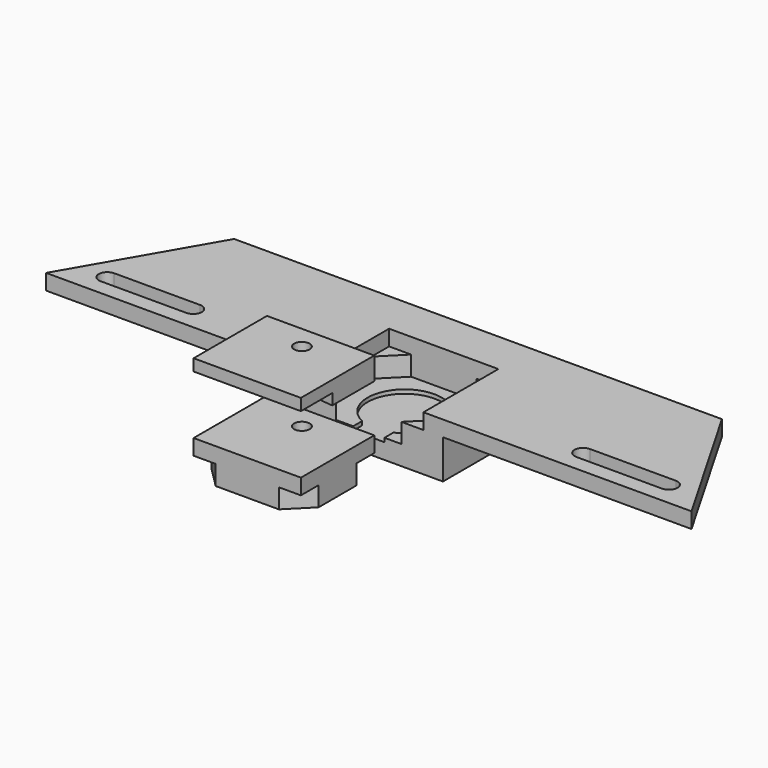
from build123d import *

# Parameters (mm, degrees)
F1_DEPTH       = 4
F3_DEPTH       = 10
F6_W           = 28
F6_H           = 24
F7_DEPTH       = 5
F8_DEPTH       = 1
F9_W           = 27.5
F9_H           = 23.5
F10_DEPTH      = 5
F10_DEPTH_BACK = 4
F11_R          = 6.5
F12_DEPTH      = 1
F14_DEPTH      = 5
F16_W          = 27.5
F16_H          = 23.5
F17_DEPTH      = 3
F17_DEPTH_BACK = 2.8
F18_R          = 2
F19_DEPTH      = 50
F21_DEPTH      = 5
F21_DEPTH_BACK = 2
F23_DEPTH      = 25


with BuildPart() as f1:
    # F0 (on Top) → F1 (new body)
    with BuildSketch(Plane.XY):
        Polygon((-14, 35), (-62.5, 35), (-82.7072594216, 0), (-62.5, 0), (-14, 0), (-14, 24), (0, 24), (0, 35), align=None)
        with BuildLine():
            ThreePointArc((-49.9685444147, 8.4), (-47.7685444147, 6.2), (-49.9685444147, 4))
            Line((-49.9685444147, 4), (-71.9685444147, 4))
            ThreePointArc((-71.9685444147, 4), (-74.1685444147, 6.2), (-71.9685444147, 8.4))
            Line((-71.9685444147, 8.4), (-49.9685444147, 8.4))
        make_face(mode=Mode.SUBTRACT)
        Polygon((14, 35), (0, 35), (0, 24), (14, 24), (14, 0), (62.5, 0), (82.7072594216, 0), (62.5, 35), align=None)
        with BuildLine():
            Line((71.9685444147, 4), (49.9685444147, 4))
            ThreePointArc((49.9685444147, 4), (47.7685444147, 6.2), (49.9685444147, 8.4))
            Line((49.9685444147, 8.4), (71.9685444147, 8.4))
            ThreePointArc((71.9685444147, 8.4), (74.1685444147, 6.2), (71.9685444147, 4))
        make_face(mode=Mode.SUBTRACT)
    extrude(amount=F1_DEPTH)

    # F2 (on face) → F3 (join)
    with BuildSketch(Plane(origin=(0, 0, 0), x_dir=(1, 0, 0), z_dir=(0, 0, -1))):
        Polygon((19, -29), (19, 0), (14, 0), (8.3431457505, 0), (14, -5.6568542495), (14, -18.3431457505), (8.3431457505, -24), (-8.3431457505, -24), (-14, -18.3431457505), (-14, -5.6568542495), (-8.3431457505, 0), (-14, 0), (-19, 0), (-19, -29), align=None)
    extrude(amount=F3_DEPTH)

    # F6 (on offset) → F7 (join)
    with BuildSketch(Plane.XY.offset(-5)):
        with Locations((0, 12)):
            Rectangle(F6_W, F6_H)
    extrude(amount=-F7_DEPTH)

    # F5 (on offset) → F8 (cut)
    with BuildSketch(Plane.XY.offset(-5)):
        with BuildLine():
            ThreePointArc((4, 2.8831560302), (8.007808689, 6.3887379249), (9.5, 11.5))
            ThreePointArc((9.5, 11.5), (-5.1112620751, 19.507808689), (-4, 2.8831560302))
            ThreePointArc((-4, 2.8831560302), (0, 2), (4, 2.8831560302))
        make_face()
        with BuildLine():
            ThreePointArc((4, 2.8831560302), (0, 2), (-4, 2.8831560302))
            Line((-4, 2.8831560302), (-4, 0))
            Line((-4, 0), (4, 0))
            Line((4, 0), (4, 2.8831560302))
        make_face()
    extrude(amount=-F8_DEPTH, mode=Mode.SUBTRACT)


with BuildPart() as f10:
    # F9 (on Top) → F10 (new body, two sides)
    with BuildSketch(Plane.XY) as f10_sk:
        with Locations((0, -27.1897088677)):
            Rectangle(F9_W, F9_H)
    extrude(amount=F10_DEPTH)
    extrude(f10_sk.sketch, amount=-F10_DEPTH_BACK)

    # F11 (on face) → F12 (join)
    with BuildSketch(Plane(origin=(0, 0, -4), x_dir=(1, 0, 0), z_dir=(0, 0, -1))):
        with Locations((0, 27.4397088677)):
            Circle(F11_R)
    extrude(amount=F12_DEPTH)

    # F13 (on face) → F14 (cut)
    with BuildSketch(Plane(origin=(0, 0, -4), x_dir=(1, 0, 0), z_dir=(0, 0, -1))):
        Polygon((8.0931457505, 15.4397088677), (13.75, 15.4397088677), (13.75, 21.0965631172), align=None)
        Polygon((8.0931457505, 38.9397088677), (13.75, 33.2828546182), (13.75, 38.9397088677), align=None)
        Polygon((-13.75, 33.2828546182), (-8.0931457505, 38.9397088677), (-13.75, 38.9397088677), align=None)
        Polygon((-13.75, 21.0965631172), (-13.75, 15.4397088677), (-8.0931457505, 15.4397088677), align=None)
    extrude(amount=-F14_DEPTH, mode=Mode.SUBTRACT)


with BuildPart() as f17:
    # F16 (on offset) → F17 (new body, two sides)
    with BuildSketch(Plane.XY.offset(20)) as f17_sk:
        with Locations((0, -27.1897088677)):
            Rectangle(F16_W, F16_H)
    extrude(amount=F17_DEPTH)
    extrude(f17_sk.sketch, amount=-F17_DEPTH_BACK)


with BuildPart() as f19_tool:
    # F18 (on face) → F19 (new body)
    with BuildSketch(Plane.XY.offset(23)):
        with Locations((0, -21.4397088677)):
            Circle(F18_R)
    extrude(amount=-F19_DEPTH)


with BuildPart() as f10_1:
    add(f10.part)

    # F19: cut by f19_tool
    add(f19_tool.part, mode=Mode.SUBTRACT)

    # F20 (on face) → F21 (cut, two sides)
    with BuildSketch(Plane(origin=(0, 0, -4), x_dir=(1, 0, 0), z_dir=(0, 0, -1))) as f21_sk:
        Polygon((-2.050493445, 24.9223529732), (-4.0413049902, 21.4052515068), (-1.9908115452, 17.9226074013), (2.050493445, 17.9570647623), (4.0413049902, 21.4741662287), (1.9908115452, 24.9568103341), align=None)
    extrude(amount=-F21_DEPTH, mode=Mode.SUBTRACT)
    extrude(f21_sk.sketch, amount=F21_DEPTH_BACK, mode=Mode.SUBTRACT)


with BuildPart() as f17_1:
    add(f17.part)

    # F19: cut by f19_tool
    add(f19_tool.part, mode=Mode.SUBTRACT)

    # F22 (on offset) → F23 (cut)
    with BuildSketch(Plane.XY.offset(20)):
        with BuildLine():
            Line((34.0421833098, -52.062548697), (42.4481494773, -37.3960475437))
            ThreePointArc((42.4481494773, -37.3960475437), (3.0553431563, -27.9863953749), (-36.838641718, -34.9724324939))
            Line((-36.838641718, -34.9724324939), (-14.8230902851, -51.8119819462))
            Line((-14.8230902851, -51.8119819462), (34.0421833098, -52.062548697))
        make_face()
    extrude(amount=-F23_DEPTH, mode=Mode.SUBTRACT)


solid = Compound([f1.part, f10_1.part, f17_1.part])
